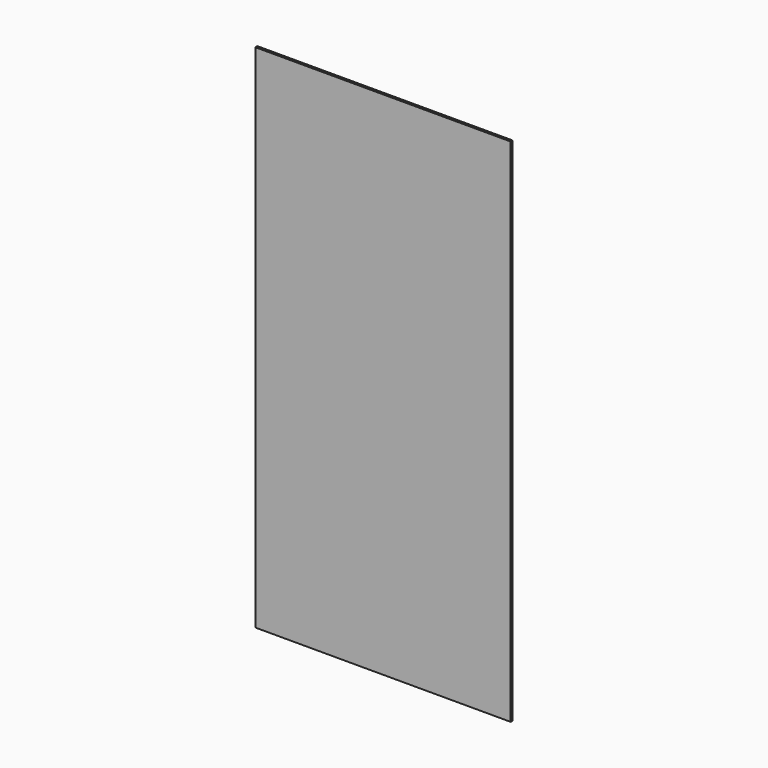
from build123d import *

# Parameters (mm, degrees)
F7_W     = 1250
F7_H     = 2500
F1_DEPTH = 12
F8_W     = 1150
F8_H     = 2400
F2_DEPTH = 200
F3_W     = 1250
F3_H     = 2500
F4_DEPTH = 12


with BuildPart() as f1:
    # F7 (on Front) → F1 (new body)
    with BuildSketch(Plane.XZ):
        Rectangle(F7_W, F7_H)
    extrude(amount=-F1_DEPTH)


with BuildPart() as f2:
    # F8 (on face) → F2 (new body)
    with BuildSketch(Plane.XZ):
        Rectangle(F8_W, F8_H)
    extrude(amount=F2_DEPTH)


with BuildPart() as f4:
    # F3 (on face) → F4 (new body)
    with BuildSketch(Plane.XZ.offset(200)):
        Rectangle(F3_W, F3_H)
    extrude(amount=F4_DEPTH)


solid = f1.part
